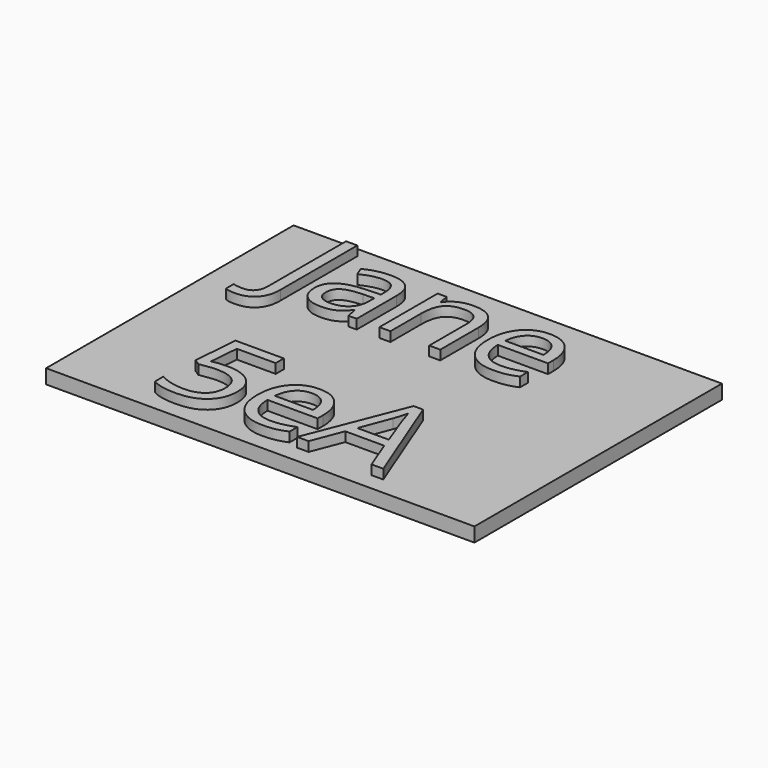
from build123d import *

# Parameters (mm, degrees)
F0_W         = 90
F0_H         = 65
F1_DEPTH     = 3
F2_TEXT_SIZE = 28.5920161407
F3_DEPTH     = 2


# Not quite as in the source:
# - Text() gives the source's letters only with a copy of the font that has no kerning and outlines rounded to 1/6400 em; it was checked with that copy


with BuildPart() as f1:
    # F0 (on Top) → F1 (new body)
    with BuildSketch(Plane.XY):
        with Locations((45, -32.5)):
            Rectangle(F0_W, F0_H)
    extrude(amount=F1_DEPTH)

    # F2 (on face) → F3 (join)
    with BuildSketch(Plane.XY.offset(3)):
        with Locations((10, -22.4489742031)):
            Text('Jane', F2_TEXT_SIZE, font='Open Sans', text_align=(TextAlign.LEFT, TextAlign.BOTTOM))
        with Locations((17.429456694, -61.3341161544)):
            Text('5eA', F2_TEXT_SIZE, font='Open Sans', text_align=(TextAlign.LEFT, TextAlign.BOTTOM))
    extrude(amount=F3_DEPTH)


solid = f1.part
